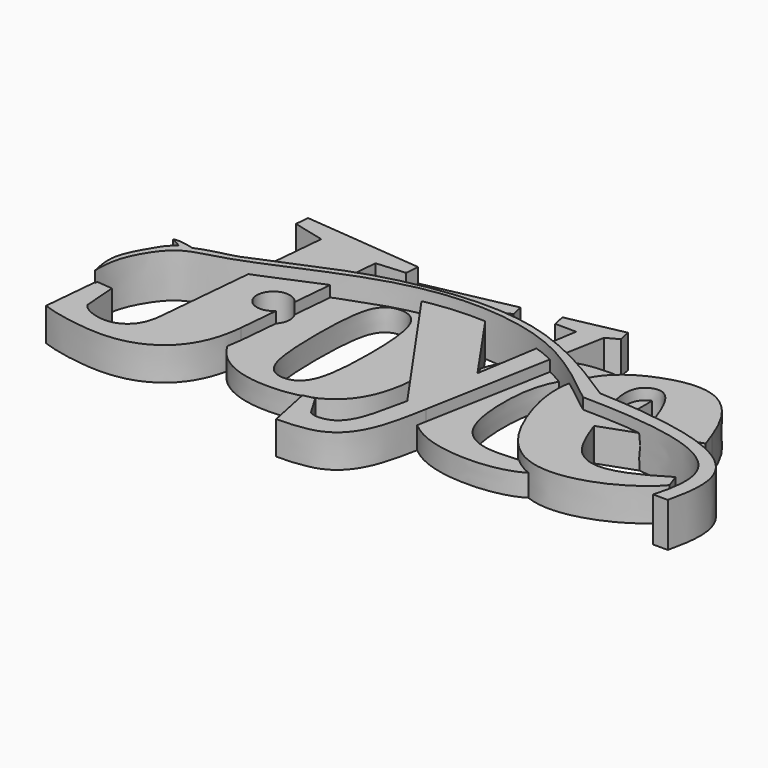
from build123d import *

# Parameters (mm, degrees)
F0_TEXT_SIZE = 34.7222222222
F5_DEPTH     = 3
F1_TEXT_SIZE = 34.7222222222
F6_DEPTH     = 2
F2_TEXT_SIZE = 34.7222222222
F7_DEPTH     = 3
F3_TEXT_SIZE = 34.7222222222
F8_DEPTH     = 2
F4_TEXT_SIZE = 34.7222222222
F9_DEPTH     = 3
F10_R        = 1.5
F11_DEPTH    = 3.0010001
F13_DEPTH    = 4


# Not quite as in the source:
# - Text() gives the source's letters only with a copy of the font that has no kerning and outlines rounded to 1/6400 em; it was checked with that copy


with BuildPart() as f5:
    # F0 (on Top) → F5 (new body)
    with BuildSketch(Plane.XY):
        with Locations(Location((-36.9728680116, -8.8983320215), (0, 0, -5.2656667278))):
            Text('J', F0_TEXT_SIZE, font='Tinos', font_style=FontStyle.BOLD, text_align=(TextAlign.LEFT, TextAlign.BOTTOM))
    extrude(amount=F5_DEPTH)

    # F1 (on Top) → F6 (join)
    with BuildSketch(Plane.XY):
        with Locations((-25.1885665537, -6.851192316)):
            Text('o', F1_TEXT_SIZE, font='Tinos', font_style=FontStyle.BOLD, text_align=(TextAlign.LEFT, TextAlign.BOTTOM))
    extrude(amount=F6_DEPTH)

    # F2 (on Top) → F7 (join)
    with BuildSketch(Plane.XY):
        with Locations(Location((-14.0746998419, -5.4125885579), (0, 0, 11.7167979564))):
            Text('y', F2_TEXT_SIZE, font='Tinos', font_style=FontStyle.BOLD, text_align=(TextAlign.LEFT, TextAlign.BOTTOM))
    extrude(amount=F7_DEPTH)

    # F3 (on Top) → F8 (join)
    with BuildSketch(Plane.XY):
        with Locations((-8.1591363678, -6.7850571051)):
            Text('c', F3_TEXT_SIZE, font='Tinos', font_style=FontStyle.BOLD, text_align=(TextAlign.LEFT, TextAlign.BOTTOM))
    extrude(amount=F8_DEPTH)

    # F4 (on Top) → F9 (join)
    with BuildSketch(Plane.XY):
        with Locations(Location((3.2775477692, -8.4646364586), (0, 0, 19.7708091249))):
            Text('e', F4_TEXT_SIZE, font='Tinos', font_style=FontStyle.BOLD, text_align=(TextAlign.LEFT, TextAlign.BOTTOM))
    extrude(amount=F9_DEPTH)

    # F10 (on face) → F11 (cut, through all)
    with BuildSketch(Plane.XY.offset(3)):
        with Locations((-23.2746042311, 1.7305533402)):
            Circle(F10_R)
    extrude(amount=-F11_DEPTH, mode=Mode.SUBTRACT)


with BuildPart() as f13:
    # F12 (on Top) → F13 (new body)
    with BuildSketch(Plane.XY):
        with BuildLine():
            add(Edge.make_bspline(
                [(17.460918054, -6.1177345924), (18.8306324805, -1.2713742132), (18.3686063475, 2.2906290483), (4.2478605644, 2.4411199109)],
                knots=[0, 0, 0, 0, 15.7428993083, 15.7428993083, 15.7428993083, 15.7428993083], degree=3))
            Line((17.460918054, -6.1177345924), (18.7947619706, -6.1177345924))
            add(Edge.make_bspline(
                [(18.7947619706, -6.1177345924), (19.8429220666, -1.428887248), (20.3299407537, 2.9793898575), (4.839187488, 3.6516441032)],
                knots=[0, 0, 0, 0, 17.0352228996, 17.0352228996, 17.0352228996, 17.0352228996], degree=3))
            add(Edge.make_bspline(
                [(4.839187488, 3.6516441032), (1.0558171944, 6.1365846185), (-6.1822112688, 10.4596164964), (-18.7630874658, 8.1761669378), (-23.2117038902, 6.0850908224), (-26.7441824165, 4.7595654566), (-28.4002282124, 3.8769350874), (-30.5497310337, 3.5281545731), (-31.6808484495, 3.0235946178)],
                knots=[0, 0, 0, 0, 0.2502263879, 0.4907673164, 0.6470767485, 0.7768740945, 0.8720078003, 1, 1, 1, 1], degree=3))
            add(Edge.make_bspline(
                [(-33.5749531418, 3.2126999657), (-32.9591949413, 3.3965279855), (-32.1041916807, 3.1223084467), (-31.6808484495, 3.0235946178)],
                knots=[0, 0, 0, 0, 1.9035213206, 1.9035213206, 1.9035213206, 1.9035213206], degree=3))
            add(Edge.make_bspline(
                [(-33.5749531418, 3.2126999657), (-33.5749531418, 3.1087791123), (-33.2035623951, 3.1158148664), (-32.6428602599, 2.692366318)],
                knots=[0, 0, 0, 0, 1.0674943772, 1.0674943772, 1.0674943772, 1.0674943772], degree=3))
            add(Edge.make_bspline(
                [(-32.6428602599, 2.692366318), (-33.3203862966, 2.228237821), (-33.8567008456, 1.2323506646), (-35.4486678097, -1.332540358), (-35.0828170483, -3.1574492775), (-34.8911433052, -4.0111177678)],
                knots=[0, 0, 0, 0, 0.2989128551, 0.6538455101, 1, 1, 1, 1], degree=3))
            add(Edge.make_bspline(
                [(4.2478605644, 2.4411199109), (2.3428034133, 3.9741851122), (-1.6368804147, 7.2098415408), (-8.0440959818, 8.8662757044), (-14.4894858348, 8.7367281404), (-21.1628219649, 6.5971794684), (-28.5201526343, 3.1361113246), (-32.1422223402, 2.5430042918), (-33.9855080792, 0.232739501), (-34.9876906338, -1.9866383911), (-34.8911433052, -4.0111177678)],
                knots=[0, 0, 0, 0, 0.1449922564, 0.2797252784, 0.4118886546, 0.5540399377, 0.7051525572, 0.8035167275, 0.8879841948, 1, 1, 1, 1], degree=3))
        make_face()
    extrude(amount=F13_DEPTH)


solid = Compound([f5.part, f13.part])
